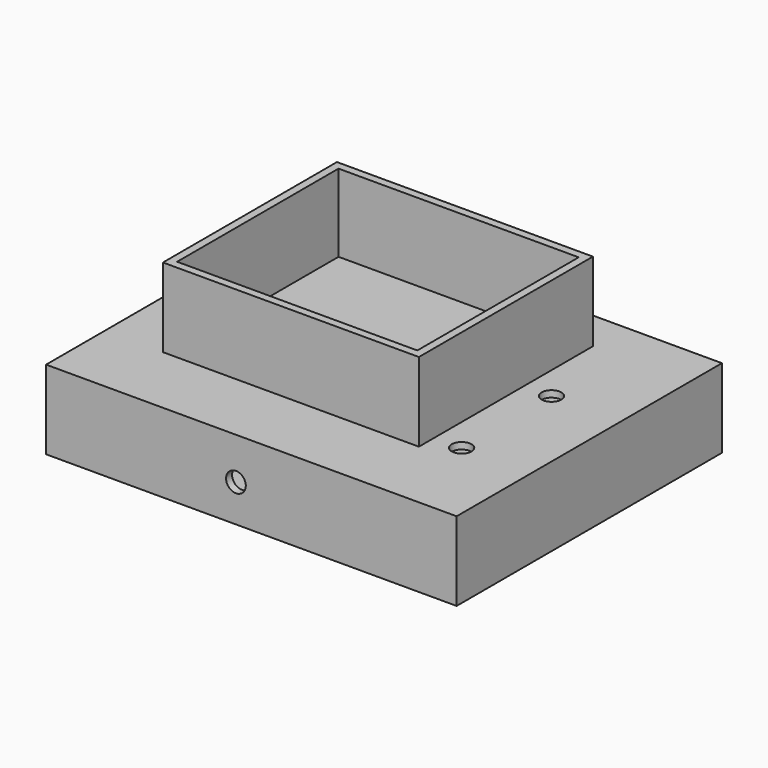
from build123d import *

# Parameters (mm, degrees)
F0_W      = 132.08
F0_H      = 106.68
F0_W_2    = 127
F0_H_2    = 101.6
F1_DEPTH  = 25.4
F2_W      = 127
F2_H      = 2.0145024173
F3_DEPTH  = 101.6
F5_D      = 6.35
F2_H_2    = 2.122098887
F6_DEPTH  = 101.6
F7_W      = 82.3423601687
F7_H      = 69.9707251042
F7_W_2    = 76.2
F7_H_2    = 63.5
F8_DEPTH  = 25.4
F10_D     = 6.35
F10_DEPTH = 12.7
F10_TIP   = 1.9077324654
F11_T     = -2.54


with BuildPart() as f1:
    # F0 (on Top) → F1 (new body)
    with BuildSketch(Plane.XY):
        with Locations((4.9622115278, -0.4122621453)):
            Rectangle(F0_W, F0_H)
        with Locations((4.3762922287, -0.5259333495)):
            Rectangle(F0_W_2, F0_H_2, mode=Mode.SUBTRACT)
    extrude(amount=F1_DEPTH)

    # F2 (on face) → F3 (join)
    with BuildSketch(Plane.XZ.offset(-50.2740666505)):
        with Locations((4.3762922287, 1.0072512086)):
            Rectangle(F2_W, F2_H)
    extrude(amount=F3_DEPTH)

    # F5 (through all)
    with Locations(Plane.XZ.offset(53.7522621453)):
        with Locations((0, 11.9956443086)):
            Hole(F5_D / 2)

    # F2 (on face) → F6 (join)
    with BuildSketch(Plane.XZ.offset(-50.2740666505)):
        with Locations((4.3762922287, 24.3389505565)):
            Rectangle(F2_W, F2_H_2)
        with Locations((4.3762922287, 1.0072512086)):
            Rectangle(F2_W, F2_H)
    extrude(amount=F6_DEPTH)

    # F7 (on face) → F8 (join)
    with BuildSketch(Plane.XY.offset(25.4)):
        with Locations((-1.2168828398, 4.8675285652)):
            Rectangle(F7_W, F7_H)
        with Locations((-1.7157470335, 5.1717488095)):
            Rectangle(F7_W_2, F7_H_2, mode=Mode.SUBTRACT)
        with Locations((-1.7157470335, 5.1717488095)):
            Rectangle(F7_W_2, F7_H_2)
    extrude(amount=F8_DEPTH)

    # F10
    with Locations(Plane.XY.offset(25.4)):
        with Locations((48.7300269306, -23.8934792578), (48.7300269306, 12.2345555574)):
            Hole(F10_D / 2, depth=F10_DEPTH)
            with Locations((0, 0, -(F10_DEPTH + F10_TIP / 2))):  # 118° drill point
                Cone(0, F10_D / 2, F10_TIP, mode=Mode.SUBTRACT)

    # F11
    f11_openings = [f1.faces().sort_by_distance(p)[0] for p in [
        (-1.216883, 4.867529, 50.8),
    ]]
    offset(amount=F11_T, openings=f11_openings)


solid = f1.part
